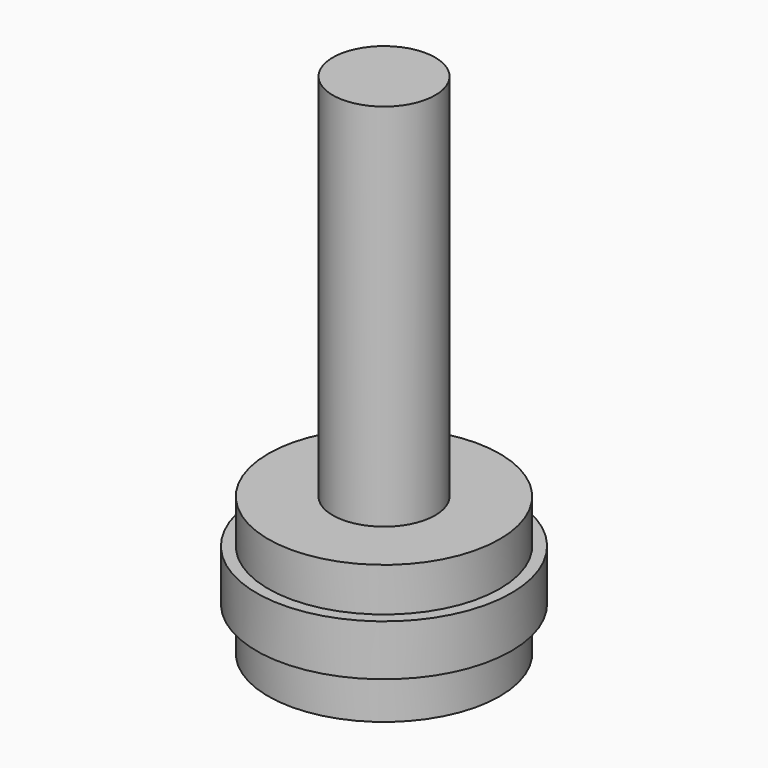
from build123d import *

# Parameters (mm, degrees)
F0_R      = 7.95
F1_DEPTH  = 3
F2_R      = 8.75
F3_DEPTH  = 3.5
F4_R      = 7.95
F5_DEPTH  = 3
F6_R      = 3
F6_R_2    = 1.05
F7_DEPTH  = 10
F10_R     = 3.51623502
F11_DEPTH = 25.4


# Not quite as in the source:
# - a feature of the source that left no trace in its solid (it failed there, or was rolled back) is left out


with BuildPart() as f1:
    # F0 (on Top) → F1 (new body)
    with BuildSketch(Plane.XY):
        with Locations((-41.0203561187, 34.5220826566)):
            Circle(F0_R)
    extrude(amount=F1_DEPTH)

    # F2 (on face) → F3 (join)
    with BuildSketch(Plane.XY.offset(3)):
        with Locations((-41.0203561187, 34.5220826566)):
            Circle(F2_R)
    extrude(amount=F3_DEPTH)

    # F4 (on face) → F5 (join)
    with BuildSketch(Plane.XY.offset(6.5)):
        with Locations((-41.0203561187, 34.5220826566)):
            Circle(F4_R)
    extrude(amount=F5_DEPTH)

    # F6 (on face) → F7 (cut)
    with BuildSketch(Plane.XY.offset(9.5)):
        with Locations((-41.0203561187, 34.5220826566)):
            Circle(F6_R)
        with Locations((-41.0203561187, 34.5220826566)):
            Circle(F6_R_2, mode=Mode.SUBTRACT)
    extrude(amount=-F7_DEPTH, mode=Mode.SUBTRACT)


with BuildPart() as f11:
    # F10 (on face) → F11 (new body)
    with BuildSketch(Plane.XY.offset(9.5)):
        with Locations((-41.0203561187, 34.5220826566)):
            Circle(F10_R)
    extrude(amount=F11_DEPTH)


solid = Compound([f1.part, f11.part])
